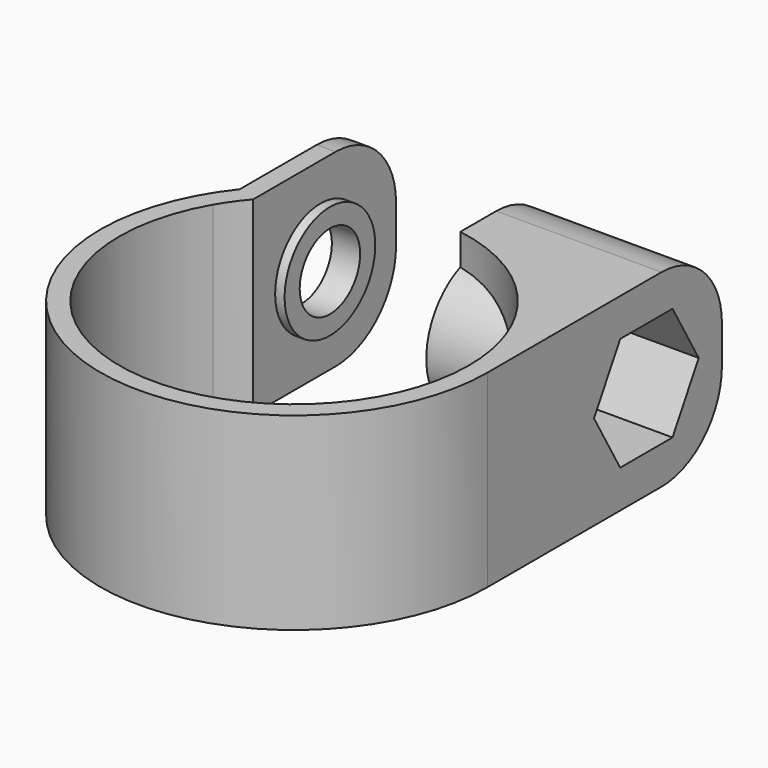
from build123d import *

# Parameters (mm, degrees)
F1_DEPTH = 20
F2_R     = 4
F3_DEPTH = 40
F2_R_2   = 6
F4_DEPTH = 3
F5_R     = 7.25
F5_R_2   = 4
F6_DEPTH = 17.5
F7_DEPTH = 12
F8_R     = 8


# Not quite as in the source:
# - a feature names something its author has since deleted; it is built from what else it names


with BuildPart() as f1:
    # F0 (on Top) → F1 (new body)
    with BuildSketch(Plane.XY):
        with BuildLine():
            Line((20.5, 0), (18.5, 0))
            ThreePointArc((18.5, 0), (-4.8088460154, -17.8640700849), (-16, 9.2870878105))
            Line((-16, 9.2870878105), (-16, 12.816005618))
            ThreePointArc((-16, 12.816005618), (-6.7915388536, -19.3423111339), (20.5, 0))
        make_face()
        with BuildLine():
            Line((-16, 31), (-16, 12.816005618))
            ThreePointArc((-16, 12.816005618), (-15.0387928923, 13.9314287976), (-14, 14.9749791319))
            Line((-14, 14.9749791319), (-14, 31))
            Line((-14, 31), (-16, 31))
        make_face()
        with BuildLine():
            Line((-16, 12.816005618), (-16, 9.2870878105))
            ThreePointArc((-16, 9.2870878105), (-15.0654846671, 10.7369069915), (-14, 12.0933866224))
            Line((-14, 12.0933866224), (-14, 14.9749791319))
            ThreePointArc((-14, 14.9749791319), (-15.0387928923, 13.9314287976), (-16, 12.816005618))
        make_face()
        with BuildLine():
            ThreePointArc((16, 12.816005618), (19.3423111339, 6.7915388536), (20.5, 0))
            Line((20.5, 0), (20.5, 31))
            Line((20.5, 31), (16, 31))
            Line((16, 31), (16, 12.816005618))
        make_face()
        with BuildLine():
            ThreePointArc((16, 9.2870878105), (17.8640700849, 4.8088460154), (18.5, 0))
            Line((18.5, 0), (20.5, 0))
            ThreePointArc((20.5, 0), (19.3423111339, 6.7915388536), (16, 12.816005618))
            Line((16, 12.816005618), (16, 9.2870878105))
        make_face()
        with BuildLine():
            ThreePointArc((3, 20.2792997907), (10.2066248083, 17.7784929064), (16, 12.816005618))
            Line((16, 12.816005618), (16, 31))
            Line((16, 31), (3, 31))
            Line((3, 31), (3, 20.2792997907))
        make_face()
        with BuildLine():
            ThreePointArc((3, 18.2551362635), (10.5050689319, 15.2280506545), (16, 9.2870878105))
            Line((16, 9.2870878105), (16, 12.816005618))
            ThreePointArc((16, 12.816005618), (10.2066248083, 17.7784929064), (3, 20.2792997907))
            Line((3, 20.2792997907), (3, 18.2551362635))
        make_face()
    extrude(amount=F1_DEPTH)

    # F2 (on face) → F3 (cut)
    with BuildSketch(Plane(origin=(-16, 0, 0), x_dir=(0, -1, 0), z_dir=(-1, 0, 0))):
        with Locations((-21, 10)):
            Circle(F2_R)
    extrude(amount=-F3_DEPTH, mode=Mode.SUBTRACT)

    # F2 (on face) → F4 (join)
    with BuildSketch(Plane(origin=(-16, 0, 0), x_dir=(0, -1, 0), z_dir=(-1, 0, 0))):
        with Locations((-21, 10)):
            Circle(F2_R_2)
        with Locations((-21, 10)):
            Circle(F2_R, mode=Mode.SUBTRACT)
    extrude(amount=-F4_DEPTH)

    # F5 (on face) → F6 (join)
    with BuildSketch(Plane.YZ.offset(20.5)):
        with Locations((21, 10)):
            Circle(F5_R)
        Polygon((14.0717967697, 10), (17.5358983849, 16), (24.4641016151, 16), (27.9282032303, 10), (24.4641016151, 4), (17.5358983849, 4), align=None, mode=Mode.SUBTRACT)
        Polygon((24.4641016151, 16), (17.5358983849, 16), (14.0717967697, 10), (17.5358983849, 4), (24.4641016151, 4), (27.9282032303, 10), align=None)
        with Locations((21, 10)):
            Circle(F5_R_2, mode=Mode.SUBTRACT)
    extrude(amount=-F6_DEPTH)

    # F5 (on face) → F7 (cut)
    with BuildSketch(Plane.YZ.offset(20.5)):
        Polygon((24.4641016151, 16), (17.5358983849, 16), (14.0717967697, 10), (17.5358983849, 4), (24.4641016151, 4), (27.9282032303, 10), align=None)
        with Locations((21, 10)):
            Circle(F5_R_2, mode=Mode.SUBTRACT)
    extrude(amount=-F7_DEPTH, mode=Mode.SUBTRACT)

    # F8
    f8_edges = [f1.edges().sort_by_distance(p)[0] for p in [
        (11.75, 31, 20),
        (-15, 31, 20),
        (11.75, 31, 0),
        (-15, 31, 0),
    ]]
    fillet(f8_edges, radius=F8_R)


solid = f1.part
